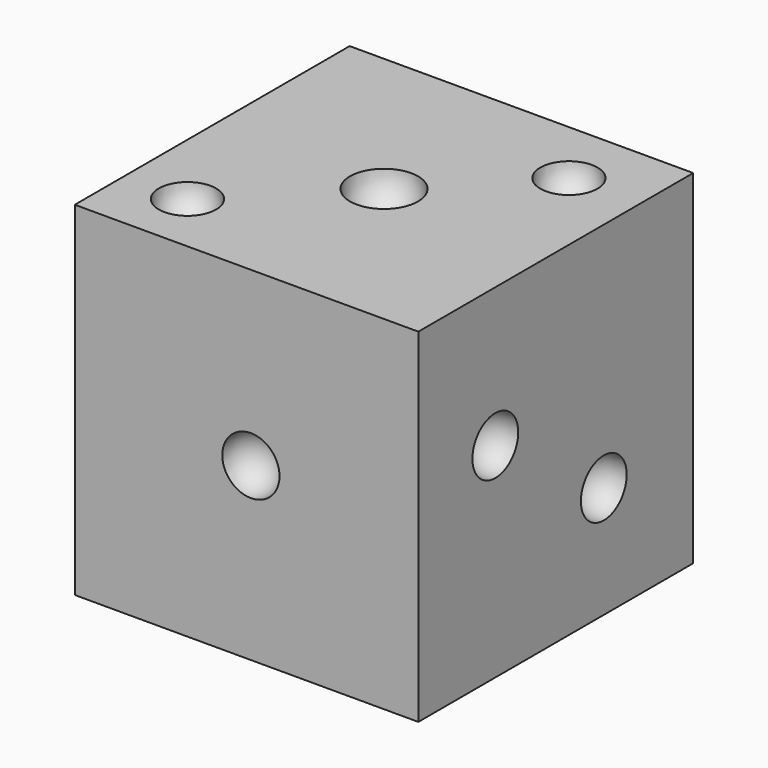
from build123d import *

# Parameters (mm, degrees)
F0_W     = 76.2
F0_H     = 76.2
F1_DEPTH = 76.2


# Not quite as in the source:
# - a feature names something its author has since deleted; it is built from what else it names


with BuildPart() as f1:
    # F0 (on Front) → F1 (new body)
    with BuildSketch(Plane.XZ):
        with Locations((38.1, 38.1)):
            Rectangle(F0_W, F0_H)
    extrude(amount=F1_DEPTH)

    # F3 (on offset) → F4 (revolve, cut)
    with BuildSketch(Plane.XZ.offset(76.2)):
        with BuildLine():
            Line((39.0552379461, 44.316590995), (39.0552379461, 31.616590995))
            ThreePointArc((39.0552379461, 31.616590995), (45.4052379461, 37.966590995), (39.0552379461, 44.316590995))
        make_face()
    revolve(axis=Axis((39.0552379461, -76.2, 38.0095466971), (0, 0, -1)), mode=Mode.SUBTRACT)

    # F6 (on face) → F7 (revolve, cut)
    with BuildSketch(Plane.YZ.offset(76.2)):
        with BuildLine():
            Line((-24.7949315235, 31.1449315235), (-24.7949315235, 18.4449315235))
            ThreePointArc((-24.7949315235, 18.4449315235), (-18.4449315235, 24.7949315235), (-24.7949315235, 31.1449315235))
        make_face()
    revolve(axis=Axis((76.2, -24.7949315235, 38.1), (0, 0, 1)), mode=Mode.SUBTRACT)

    # F8 (on face) → F9 (revolve, cut)
    with BuildSketch(Plane.YZ.offset(76.2)):
        with BuildLine():
            ThreePointArc((-54.8643916845, 38.9347406268), (-48.5143916845, 45.2847406268), (-54.8643916845, 51.6347406268))
            Line((-54.8643916845, 51.6347406268), (-54.8643916845, 38.9347406268))
        make_face()
    revolve(axis=Axis((76.2, -54.8643916845, 38.1), (0, 0, -1)), mode=Mode.SUBTRACT)

    # F5 (on face) → F10 (revolve, cut)
    with BuildSketch(Plane.XY.offset(76.2)):
        with BuildLine():
            ThreePointArc((13.884774404, -68.665225596), (20.234774404, -62.315225596), (13.884774404, -55.965225596))
            Line((13.884774404, -55.965225596), (13.884774404, -68.665225596))
        make_face()
    revolve(axis=Axis((13.884774404, -38.1, 76.2), (0, -1, 0)), mode=Mode.SUBTRACT)

    # F11 (on face) → F12 (revolve, cut)
    with BuildSketch(Plane.XY.offset(76.2)):
        with BuildLine():
            ThreePointArc((60.6395359006, -21.2940271984), (66.9406648647, -14.8955294233), (60.5421670896, -8.5944004593))
            Line((60.5421670896, -8.5944004593), (60.6395359006, -21.2940271984))
        make_face()
    revolve(axis=Axis((60.7683883168, -38.1, 76.2), (0.0076668355, -0.9999706094, 0)), mode=Mode.SUBTRACT)

    # F13 (on face) → F14 (revolve, cut)
    with BuildSketch(Plane.XY.offset(76.2)):
        with BuildLine():
            ThreePointArc((38.1, -45.6513431721), (45.6513431721, -38.1), (38.1, -30.5486568279))
            Line((38.1, -30.5486568279), (38.1, -45.6513431721))
        make_face()
    revolve(axis=Axis((38.1, -38.1, 76.2), (0, -1, 0)), mode=Mode.SUBTRACT)

    # F15 (on face) → F16 (revolve, cut)
    with BuildSketch(Plane(origin=(0, 0, 0), x_dir=(0, -1, 0), z_dir=(-1, 0, 0))):
        with BuildLine():
            ThreePointArc((62.3152181506, 1.1483397499), (68.6652181506, 7.4983397499), (62.3152181506, 13.8483397499))
            Line((62.3152181506, 13.8483397499), (62.3152181506, 1.1483397499))
        make_face()
        with BuildLine():
            ThreePointArc((62.3152181506, 62.3516621232), (68.6652181506, 68.7016621232), (62.3152181506, 75.0516621232))
            Line((62.3152181506, 75.0516621232), (62.3152181506, 62.3516621232))
        make_face()
    revolve(axis=Axis((0, -62.3152181506, 38.1), (0, 0, -1)), mode=Mode.SUBTRACT)

    # F17 (on face) → F18 (revolve, cut)
    with BuildSketch(Plane(origin=(0, 0, 0), x_dir=(0, -1, 0), z_dir=(-1, 0, 0))):
        with BuildLine():
            Line((12.2881568968, 71.8361058897), (12.2881568968, 59.1807892852))
            ThreePointArc((12.2881568968, 59.1807892852), (18.1059535429, 65.5084475875), (12.2881568968, 71.8361058897))
        make_face()
        with BuildLine():
            ThreePointArc((12.2881568968, 2.2350881555), (18.1059535429, 8.5627464578), (12.2881568968, 14.89040476))
            Line((12.2881568968, 14.89040476), (12.2881568968, 2.2350881555))
        make_face()
    revolve(axis=Axis((0, -12.2881568968, 39.2175440778), (0, 0, -1)), mode=Mode.SUBTRACT)

    # F19 (on face) → F20 (revolve, cut)
    with BuildSketch(Plane(origin=(0, 0, 0), x_dir=(-1, 0, 0), z_dir=(0, 1, 0))):
        with BuildLine():
            ThreePointArc((-38.1, 31.75), (-31.75, 38.1), (-38.1, 44.45))
            Line((-38.1, 44.45), (-38.1, 31.75))
        make_face()
    revolve(axis=Axis((38.1, 0, 38.1), (0, 0, -1)), mode=Mode.SUBTRACT)

    # F21 (on face) → F22 (revolve, cut)
    with BuildSketch(Plane(origin=(0, 0, 0), x_dir=(-1, 0, 0), z_dir=(0, 1, 0))):
        with BuildLine():
            ThreePointArc((-59.0270198882, 50.5481952965), (-52.6770198882, 56.8981952965), (-59.0270198882, 63.2481952965))
            Line((-59.0270198882, 63.2481952965), (-59.0270198882, 50.5481952965))
        make_face()
        with BuildLine():
            ThreePointArc((-59.0270198882, 11.1651918083), (-52.6770198882, 17.5151918083), (-59.0270198882, 23.8651918083))
            Line((-59.0270198882, 23.8651918083), (-59.0270198882, 11.1651918083))
        make_face()
    revolve(axis=Axis((59.0270198882, 0, 38.1), (0, 0, -1)), mode=Mode.SUBTRACT)

    # F23 (on face) → F24 (revolve, cut)
    with BuildSketch(Plane(origin=(0, 0, 0), x_dir=(-1, 0, 0), z_dir=(0, 1, 0))):
        with BuildLine():
            ThreePointArc((-16.450792551, 50.5481952965), (-10.100792551, 56.8981952965), (-16.450792551, 63.2481952965))
            Line((-16.450792551, 63.2481952965), (-16.450792551, 50.5481952965))
        make_face()
        with BuildLine():
            ThreePointArc((-16.450792551, 11.1651918083), (-10.100792551, 17.5151918083), (-16.450792551, 23.8651918083))
            Line((-16.450792551, 23.8651918083), (-16.450792551, 11.1651918083))
        make_face()
    revolve(axis=Axis((16.450792551, 0, 38.1), (0, 0, -1)), mode=Mode.SUBTRACT)

    # F25 (on face) → F26 (revolve, cut)
    with BuildSketch(Plane(origin=(0, 0, 0), x_dir=(1, 0, 0), z_dir=(0, 0, -1))):
        with BuildLine():
            ThreePointArc((20.2712118626, 53.3042097628), (26.6212118626, 59.6542097628), (20.2712118626, 66.0042097628))
            Line((20.2712118626, 66.0042097628), (20.2712118626, 53.3042097628))
        make_face()
        with BuildLine():
            ThreePointArc((20.2712118626, 27.7584748507), (26.6212118626, 34.1084748507), (20.2712118626, 40.4584748507))
            Line((20.2712118626, 40.4584748507), (20.2712118626, 27.7584748507))
        make_face()
        with BuildLine():
            Line((20.2712118626, 18.6381624848), (20.2712118626, 5.9381624848))
            ThreePointArc((20.2712118626, 5.9381624848), (26.6212118626, 12.2881624848), (20.2712118626, 18.6381624848))
        make_face()
    revolve(axis=Axis((20.2712118626, -38.1, 0), (0, 1, 0)), mode=Mode.SUBTRACT)

    # F27 (on face) → F28 (revolve, cut)
    with BuildSketch(Plane(origin=(0, 0, 0), x_dir=(1, 0, 0), z_dir=(0, 0, -1))):
        with BuildLine():
            ThreePointArc((49.5423637331, 52.2398049176), (55.8923637331, 58.5898049176), (49.5423637331, 64.9398049176))
            Line((49.5423637331, 64.9398049176), (49.5423637331, 52.2398049176))
        make_face()
        with BuildLine():
            ThreePointArc((49.5423637331, 31.75), (55.8923637331, 38.1), (49.5423637331, 44.45))
            Line((49.5423637331, 44.45), (49.5423637331, 31.75))
        make_face()
        with BuildLine():
            Line((49.5423637331, 20.2347697526), (49.5423637331, 7.5347697526))
            ThreePointArc((49.5423637331, 7.5347697526), (55.8923637331, 13.8847697526), (49.5423637331, 20.2347697526))
        make_face()
    revolve(axis=Axis((49.5423637331, -38.1, 0), (0, 1, 0)), mode=Mode.SUBTRACT)


solid = f1.part
